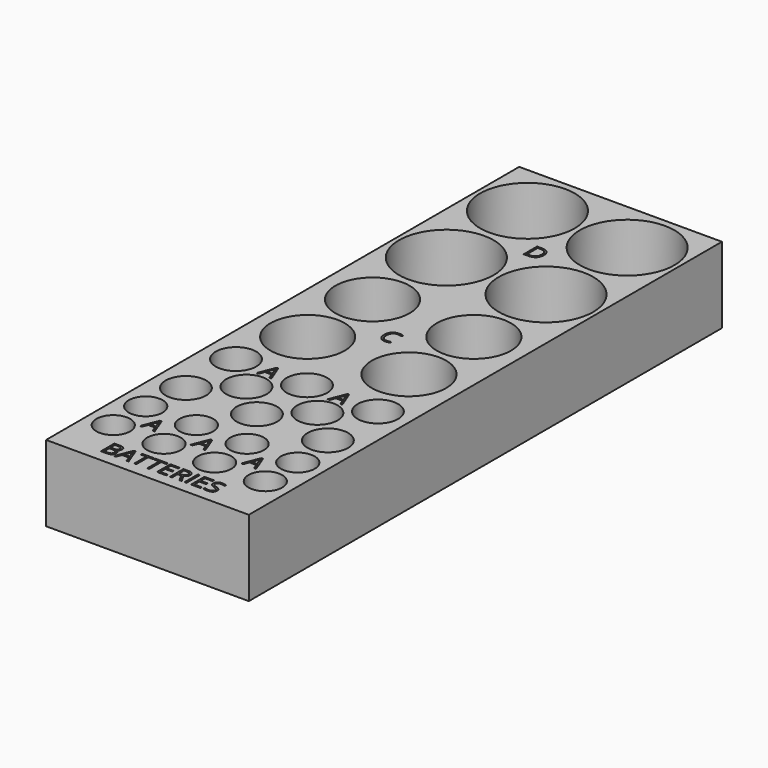
from build123d import *

# Parameters (mm, degrees)
F0_W         = 76.2
F0_H         = 260.35
F0_R         = 6.35
F0_R_2       = 7.62
F0_R_3       = 13.97
F0_R_4       = 17.78
F1_DEPTH     = 25.4
F2_TEXT_SIZE = 8.8194444444
F3_DEPTH     = 1.5875
F4_W         = 76.2
F4_H         = 38.1
F5_DEPTH     = 25.401
F7_W         = 76.2
F7_H         = 222.25
F8_DEPTH     = 3.175


# Not quite as in the source:
# - Text() gives the source's letters only with a copy of the font that has no kerning and outlines rounded to 1/6400 em; it was checked with that copy


with BuildPart() as f1:
    # F0 (on Top) → F1 (new body)
    with BuildSketch(Plane.XY):
        Rectangle(F0_W, F0_H)
        with Locations((-28.575, -72.4142592165)):
            Circle(F0_R, mode=Mode.SUBTRACT)
        with Locations((-9.525, -72.4142592165)):
            Circle(F0_R, mode=Mode.SUBTRACT)
        with Locations((-28.575, -57.1742592165)):
            Circle(F0_R, mode=Mode.SUBTRACT)
        with Locations((-26.67, -40.6642592165)):
            Circle(F0_R_2, mode=Mode.SUBTRACT)
        with Locations((-26.67, -17.1435300611)):
            Circle(F0_R_2, mode=Mode.SUBTRACT)
        with Locations((-9.525, -57.1742592165)):
            Circle(F0_R, mode=Mode.SUBTRACT)
        with Locations((-13.335, -28.9038946388)):
            Circle(F0_R_2, mode=Mode.SUBTRACT)
        with Locations((9.525, -72.4142592165)):
            Circle(F0_R, mode=Mode.SUBTRACT)
        with Locations((28.575, -72.4142592165)):
            Circle(F0_R, mode=Mode.SUBTRACT)
        with Locations((0, -40.6642592165)):
            Circle(F0_R_2, mode=Mode.SUBTRACT)
        with Locations((9.525, -57.1742592165)):
            Circle(F0_R, mode=Mode.SUBTRACT)
        with Locations((0, -17.1435300611)):
            Circle(F0_R_2, mode=Mode.SUBTRACT)
        with Locations((13.335, -28.9038946388)):
            Circle(F0_R_2, mode=Mode.SUBTRACT)
        with Locations((26.67, -40.6642592165)):
            Circle(F0_R_2, mode=Mode.SUBTRACT)
        with Locations((28.575, -57.1742592165)):
            Circle(F0_R, mode=Mode.SUBTRACT)
        with Locations((26.67, -17.1435300611)):
            Circle(F0_R_2, mode=Mode.SUBTRACT)
        with Locations((-19.05, 6.9864699389)):
            Circle(F0_R_3, mode=Mode.SUBTRACT)
        with Locations((-19.05, 37.4664699389)):
            Circle(F0_R_3, mode=Mode.SUBTRACT)
        with Locations((-18.7325, 71.755)):
            Circle(F0_R_4, mode=Mode.SUBTRACT)
        with Locations((-18.7325, 109.855)):
            Circle(F0_R_4, mode=Mode.SUBTRACT)
        with Locations((19.05, 6.9864699389)):
            Circle(F0_R_3, mode=Mode.SUBTRACT)
        with Locations((19.05, 37.4664699389)):
            Circle(F0_R_3, mode=Mode.SUBTRACT)
        with Locations((18.7325, 71.755)):
            Circle(F0_R_4, mode=Mode.SUBTRACT)
        with Locations((18.7325, 109.855)):
            Circle(F0_R_4, mode=Mode.SUBTRACT)
    extrude(amount=F1_DEPTH)

    # F2 (on face) → F3 (cut)
    with BuildSketch(Plane.XY.offset(25.4)):
        with Locations((-3.231499566, 87.63)):
            Text('D', F2_TEXT_SIZE, font='Open Sans', text_align=(TextAlign.LEFT, TextAlign.BOTTOM))
        with Locations((-2.9365993924, 19.0514699389)):
            Text('C', F2_TEXT_SIZE, font='Open Sans', text_align=(TextAlign.LEFT, TextAlign.BOTTOM))
        with Locations((-16.4114702691, -20.3185300611)):
            Text('A', F2_TEXT_SIZE, font='Open Sans', text_align=(TextAlign.LEFT, TextAlign.BOTTOM))
        with Locations((10.2585297309, -20.3185300611)):
            Text('A', F2_TEXT_SIZE, font='Open Sans', text_align=(TextAlign.LEFT, TextAlign.BOTTOM))
        with Locations((-22.1264702691, -67.9692592165)):
            Text('A', F2_TEXT_SIZE, font='Open Sans', text_align=(TextAlign.LEFT, TextAlign.BOTTOM))
        with Locations((-3.0764702691, -67.9692592165)):
            Text('A', F2_TEXT_SIZE, font='Open Sans', text_align=(TextAlign.LEFT, TextAlign.BOTTOM))
        with Locations((15.9735297309, -67.9692592165)):
            Text('A', F2_TEXT_SIZE, font='Open Sans', text_align=(TextAlign.LEFT, TextAlign.BOTTOM))
        with Locations((-21.8818714, -87.6542592165)):
            Text('BATTERIES', F2_TEXT_SIZE, font='Open Sans', text_align=(TextAlign.LEFT, TextAlign.BOTTOM))
    extrude(amount=-F3_DEPTH, mode=Mode.SUBTRACT)

    # F4 (on face) → F5 (cut, through all)
    with BuildSketch(Plane.XY.offset(25.4)):
        with Locations((0, -111.125)):
            Rectangle(F4_W, F4_H)
    extrude(amount=-F5_DEPTH, mode=Mode.SUBTRACT)

    # F7 (on face) → F8 (join)
    with BuildSketch(Plane(origin=(0, 0, 0), x_dir=(1, 0, 0), z_dir=(0, 0, -1))):
        with Locations((0, -19.05)):
            Rectangle(F7_W, F7_H)
    extrude(amount=F8_DEPTH)


solid = f1.part
